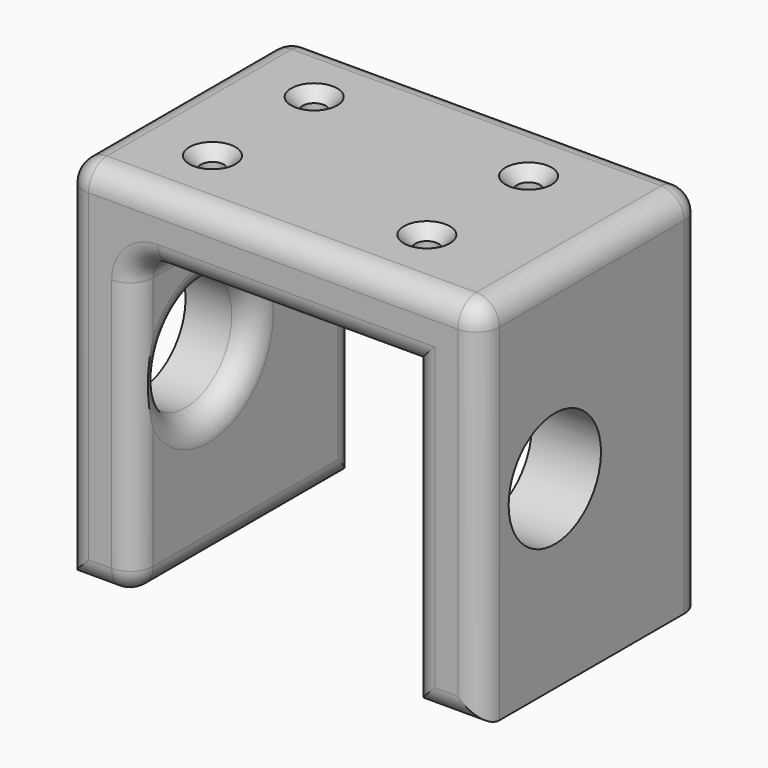
from build123d import *

# Parameters (mm, degrees)
F1_DEPTH       = 38.1
F3_D           = 31.75
F4_T1_DEPTH    = 76.2
F4_T3_DEPTH    = 101.6
F4_T5_DEPTH    = 111.125
F4_T7_DEPTH    = 28.575
F4_T9_DEPTH    = 69.85
F4_T11_DEPTH   = 69.85
F4_T13_DEPTH   = 98.425
F4_T15_DEPTH   = 50.8
F4_T17_DEPTH   = 63.5
F4_T19_DEPTH   = 85.725
F4_T21_DEPTH   = 92.075
F4_S25_W       = 6.477
F4_S25_H       = 6.477
F4_T26_DEPTH   = 6.477
F4_S31_W       = 6.477
F4_S31_H       = 6.477
F4_T32_DEPTH   = 6.477
F4_S37_W       = 6.477
F4_S37_H       = 6.477
F4_T38_DEPTH   = 6.477
F4_S43_W       = 6.477
F4_S43_H       = 6.477
F4_T44_DEPTH   = 6.477
F4_S49_W       = 6.477
F4_S49_H       = 6.477
F4_T50_DEPTH   = 6.477
F4_T56_ANGLE   = 90
F4_T58_ANGLE   = 90
F4_T63_DEPTH   = 85.725
F4_T67_DEPTH   = 98.425
F4_T74_DEPTH   = 85.725
F4_T78_DEPTH   = 98.425
F6_D           = 6.35
F6_DEPTH       = 12.7
F6_CSINK_D     = 12.7
F6_CSINK_ANGLE = 90
F6_TIP         = 1.9077324654


# Not quite as in the source:
# - a fillet or chamfer that OpenCascade refuses, or shapes differently, is made with other operations: its cross-section is extruded or revolved along the edge and cut away or added


with BuildPart() as f1:
    # F0 (on Front) → F1 (new body, symmetric)
    with BuildSketch(Plane.XZ):
        Polygon((57.15, 50.8), (-57.15, 50.8), (-57.15, -50.8), (-38.1, -50.8), (-38.1, 31.75), (38.1, 31.75), (38.1, -50.8), (57.15, -50.8), align=None)
    extrude(amount=F1_DEPTH, both=True)

    # F3 (through all)
    with Locations(Plane.YZ.offset(57.15)):
        with Locations((-12.7, 0)):
            Hole(F3_D / 2)

    # F4: fillet of radius 6.35 on 19 edges, made by hand

    # F4_s2 → F4_t1 (join)
    with BuildSketch(Plane.XZ.offset(-38.1)):
        with BuildLine():
            ThreePointArc((-38.1, 25.4), (-36.2401280605, 29.8901280605), (-31.75, 31.75))
            Line((-31.75, 31.75), (-38.1, 31.75))
            Line((-38.1, 31.75), (-38.1, 25.4))
        make_face()
    extrude(amount=F4_T1_DEPTH)

    # F4_s4 → F4_t3 (cut)
    with BuildSketch(Plane.YZ.offset(-50.8)):
        with BuildLine():
            ThreePointArc((-31.75, 50.8), (-36.2401280605, 48.9401280605), (-38.1, 44.45))
            Line((-38.1, 44.45), (-38.1, 50.8))
            Line((-38.1, 50.8), (-31.75, 50.8))
        make_face()
        with BuildLine():
            ThreePointArc((31.75, 50.8), (36.2401280605, 48.9401280605), (38.1, 44.45))
            Line((38.1, 44.45), (38.1, 50.8))
            Line((38.1, 50.8), (31.75, 50.8))
        make_face()
    extrude(amount=F4_T3_DEPTH, mode=Mode.SUBTRACT)

    # F4_s6 → F4_t5 (cut)
    with BuildSketch(Plane.XY.offset(-66.675)):
        with BuildLine():
            ThreePointArc((-57.15, -31.75), (-55.2901280605, -36.2401280605), (-50.8, -38.1))
            Line((-50.8, -38.1), (-57.15, -38.1))
            Line((-57.15, -38.1), (-57.15, -31.75))
        make_face()
        with BuildLine():
            ThreePointArc((50.8, -38.1), (55.2901280605, -36.2401280605), (57.15, -31.75))
            Line((57.15, -31.75), (57.15, -38.1))
            Line((57.15, -38.1), (50.8, -38.1))
        make_face()
        with BuildLine():
            ThreePointArc((50.8, 38.1), (55.2901280605, 36.2401280605), (57.15, 31.75))
            Line((57.15, 31.75), (57.15, 38.1))
            Line((57.15, 38.1), (50.8, 38.1))
        make_face()
        with BuildLine():
            ThreePointArc((-50.8, 38.1), (-55.2901280605, 36.2401280605), (-57.15, 31.75))
            Line((-57.15, 31.75), (-57.15, 38.1))
            Line((-57.15, 38.1), (-50.8, 38.1))
        make_face()
    extrude(amount=F4_T5_DEPTH, mode=Mode.SUBTRACT)

    # F4_s8 → F4_t7 (cut)
    with BuildSketch(Plane.YZ.offset(-73.025)):
        with BuildLine():
            ThreePointArc((-38.1, -44.45), (-36.2401280605, -48.9401280605), (-31.75, -50.8))
            Line((-31.75, -50.8), (-38.1, -50.8))
            Line((-38.1, -50.8), (-38.1, -44.45))
        make_face()
    extrude(amount=F4_T7_DEPTH, mode=Mode.SUBTRACT)

    # F4_s10 → F4_t9 (cut)
    with BuildSketch(Plane.XY.offset(-44.45)):
        with BuildLine():
            ThreePointArc((-44.45, -38.1), (-39.9598719395, -36.2401280605), (-38.1, -31.75))
            Line((-38.1, -31.75), (-38.1, -38.1))
            Line((-38.1, -38.1), (-44.45, -38.1))
        make_face()
    extrude(amount=F4_T9_DEPTH, mode=Mode.SUBTRACT)

    # F4_s12 → F4_t11 (cut)
    with BuildSketch(Plane.YZ.offset(-31.75)):
        with BuildLine():
            ThreePointArc((-38.1, 38.1), (-36.2401280605, 33.6098719395), (-31.75, 31.75))
            Line((-31.75, 31.75), (-38.1, 31.75))
            Line((-38.1, 31.75), (-38.1, 38.1))
        make_face()
        with BuildLine():
            ThreePointArc((38.1, 38.1), (36.2401280605, 33.6098719395), (31.75, 31.75))
            Line((31.75, 31.75), (38.1, 31.75))
            Line((38.1, 31.75), (38.1, 38.1))
        make_face()
    extrude(amount=F4_T11_DEPTH, mode=Mode.SUBTRACT)

    # F4_s14 → F4_t13 (cut)
    with BuildSketch(Plane.XY.offset(-66.675)):
        with BuildLine():
            ThreePointArc((44.45, -38.1), (39.9598719395, -36.2401280605), (38.1, -31.75))
            Line((38.1, -31.75), (38.1, -38.1))
            Line((38.1, -38.1), (44.45, -38.1))
        make_face()
        with BuildLine():
            ThreePointArc((44.45, 38.1), (39.9598719395, 36.2401280605), (38.1, 31.75))
            Line((38.1, 31.75), (38.1, 38.1))
            Line((38.1, 38.1), (44.45, 38.1))
        make_face()
    extrude(amount=F4_T13_DEPTH, mode=Mode.SUBTRACT)

    # F4_s16 → F4_t15 (cut)
    with BuildSketch(Plane.YZ.offset(22.225)):
        with BuildLine():
            ThreePointArc((-38.1, -44.45), (-36.2401280605, -48.9401280605), (-31.75, -50.8))
            Line((-31.75, -50.8), (-38.1, -50.8))
            Line((-38.1, -50.8), (-38.1, -44.45))
        make_face()
    extrude(amount=F4_T15_DEPTH, mode=Mode.SUBTRACT)

    # F4_s18 → F4_t17 (cut)
    with BuildSketch(Plane.XZ.offset(-31.75)):
        with BuildLine():
            ThreePointArc((-50.8, 50.8), (-55.2901280605, 48.9401280605), (-57.15, 44.45))
            Line((-57.15, 44.45), (-57.15, 50.8))
            Line((-57.15, 50.8), (-50.8, 50.8))
        make_face()
        with BuildLine():
            ThreePointArc((50.8, 50.8), (55.2901280605, 48.9401280605), (57.15, 44.45))
            Line((57.15, 44.45), (57.15, 50.8))
            Line((57.15, 50.8), (50.8, 50.8))
        make_face()
    extrude(amount=F4_T17_DEPTH, mode=Mode.SUBTRACT)

    # F4_s20 → F4_t19 (cut)
    with BuildSketch(Plane.XZ.offset(-53.975)):
        with BuildLine():
            ThreePointArc((-44.45, -50.8), (-39.9598719395, -48.9401280605), (-38.1, -44.45))
            Line((-38.1, -44.45), (-38.1, -50.8))
            Line((-38.1, -50.8), (-44.45, -50.8))
        make_face()
    extrude(amount=F4_T19_DEPTH, mode=Mode.SUBTRACT)

    # F4_s22 → F4_t21 (cut)
    with BuildSketch(Plane.XY.offset(-66.675)):
        with BuildLine():
            ThreePointArc((-44.45, 38.1), (-39.9598719395, 36.2401280605), (-38.1, 31.75))
            Line((-38.1, 31.75), (-38.1, 38.1))
            Line((-38.1, 38.1), (-44.45, 38.1))
        make_face()
    extrude(amount=F4_T21_DEPTH, mode=Mode.SUBTRACT)


with BuildPart() as f4_tool24:
    # F4_s25 → F4_t26 (new body)
    with BuildSketch(Plane.XY.offset(44.45)):
        with Locations((54.0385, -34.9885)):
            Rectangle(F4_S25_W, F4_S25_H)
    extrude(amount=F4_T26_DEPTH)

    # F4_s27 → F4_t28 (revolve, cut)
    with BuildSketch(Plane(origin=(50.8, -31.75, 44.45), x_dir=(-0.7071067812, 0.7071067812, 0), z_dir=(0.7071067812, 0.7071067812, 0))):
        with BuildLine():
            ThreePointArc((0, -6.35), (6.35, 0), (0, 6.35))
            Line((0, 6.35), (0, -6.35))
        make_face()
    revolve(axis=Axis((50.8, -31.75, 44.45), (0, 0, 1)), mode=Mode.SUBTRACT)


with BuildPart() as f1_1:
    add(f1.part)

    # F4_t23: cut F4_tool24
    add(f4_tool24.part, mode=Mode.SUBTRACT)


with BuildPart() as f4_tool30:
    # F4_s31 → F4_t32 (new body)
    with BuildSketch(Plane.XY.offset(44.45)):
        with Locations((-54.0385, -34.9885)):
            Rectangle(F4_S31_W, F4_S31_H)
    extrude(amount=F4_T32_DEPTH)

    # F4_s33 → F4_t34 (revolve, cut)
    with BuildSketch(Plane(origin=(-50.8, -31.75, 44.45), x_dir=(0.7071067812, 0.7071067812, 0), z_dir=(0.7071067812, -0.7071067812, 0))):
        with BuildLine():
            ThreePointArc((0, -6.35), (6.35, 0), (0, 6.35))
            Line((0, 6.35), (0, -6.35))
        make_face()
    revolve(axis=Axis((-50.8, -31.75, 44.45), (0, 0, 1)), mode=Mode.SUBTRACT)


with BuildPart() as f1_2:
    add(f1_1.part)

    # F4_t29: cut F4_tool30
    add(f4_tool30.part, mode=Mode.SUBTRACT)


with BuildPart() as f4_tool36:
    # F4_s37 → F4_t38 (new body)
    with BuildSketch(Plane.XZ.offset(31.75)):
        with Locations((-41.2115, -47.6885)):
            Rectangle(F4_S37_W, F4_S37_H)
    extrude(amount=F4_T38_DEPTH)

    # F4_s39 → F4_t40 (revolve, cut)
    with BuildSketch(Plane(origin=(-44.45, -31.75, -44.45), x_dir=(-0.7071067812, 0, 0.7071067812), z_dir=(0.7071067812, 0, 0.7071067812))):
        with BuildLine():
            ThreePointArc((0, -6.35), (6.35, 0), (0, 6.35))
            Line((0, 6.35), (0, -6.35))
        make_face()
    revolve(axis=Axis((-44.45, -31.75, -44.45), (0, -1, 0)), mode=Mode.SUBTRACT)


with BuildPart() as f1_3:
    add(f1_2.part)

    # F4_t35: cut F4_tool36
    add(f4_tool36.part, mode=Mode.SUBTRACT)


with BuildPart() as f4_tool42:
    # F4_s43 → F4_t44 (new body)
    with BuildSketch(Plane.XY.offset(44.45)):
        with Locations((-54.0385, 34.9885)):
            Rectangle(F4_S43_W, F4_S43_H)
    extrude(amount=F4_T44_DEPTH)

    # F4_s45 → F4_t46 (revolve, cut)
    with BuildSketch(Plane(origin=(-50.8, 31.75, 44.45), x_dir=(0.7071067812, -0.7071067812, 0), z_dir=(-0.7071067812, -0.7071067812, 0))):
        with BuildLine():
            ThreePointArc((0, -6.35), (6.35, 0), (0, 6.35))
            Line((0, 6.35), (0, -6.35))
        make_face()
    revolve(axis=Axis((-50.8, 31.75, 44.45), (0, 0, 1)), mode=Mode.SUBTRACT)


with BuildPart() as f1_4:
    add(f1_3.part)

    # F4_t41: cut F4_tool42
    add(f4_tool42.part, mode=Mode.SUBTRACT)


with BuildPart() as f4_tool48:
    # F4_s49 → F4_t50 (new body)
    with BuildSketch(Plane.XY.offset(44.45)):
        with Locations((54.0385, 34.9885)):
            Rectangle(F4_S49_W, F4_S49_H)
    extrude(amount=F4_T50_DEPTH)

    # F4_s51 → F4_t52 (revolve, cut)
    with BuildSketch(Plane(origin=(50.8, 31.75, 44.45), x_dir=(-0.7071067812, -0.7071067812, 0), z_dir=(-0.7071067812, 0.7071067812, 0))):
        with BuildLine():
            ThreePointArc((0, -6.35), (6.35, 0), (0, 6.35))
            Line((0, 6.35), (0, -6.35))
        make_face()
    revolve(axis=Axis((50.8, 31.75, 44.45), (0, 0, 1)), mode=Mode.SUBTRACT)


with BuildPart() as f1_5:
    add(f1_4.part)

    # F4_t47: cut F4_tool48
    add(f4_tool48.part, mode=Mode.SUBTRACT)

    # F4_s53 → F4_t54 (revolve, cut)
    with BuildSketch(Plane.XY):
        with BuildLine():
            ThreePointArc((-38.1, 9.525), (-39.9598719395, 5.0348719395), (-44.45, 3.175))
            Line((-44.45, 3.175), (-38.1, 3.175))
            Line((-38.1, 3.175), (-38.1, 9.525))
        make_face()
    revolve(axis=Axis((-38.1, -12.7, 0), (1, 0, 0)), mode=Mode.SUBTRACT)

    # F4_s55 → F4_t56 (revolve, cut)
    with BuildSketch(Plane.XY.offset(25.4)):
        with BuildLine():
            ThreePointArc((-44.45, 38.1), (-39.9598719395, 36.2401280605), (-38.1, 31.75))
            Line((-38.1, 31.75), (-38.1, 38.1))
            Line((-38.1, 38.1), (-44.45, 38.1))
        make_face()
    revolve(axis=Axis((-31.75, 38.1, 25.4), (0, 1, 0)), revolution_arc=F4_T56_ANGLE, mode=Mode.SUBTRACT)

    # F4_s57 → F4_t58 (revolve, cut)
    with BuildSketch(Plane.XY.offset(25.4)):
        with BuildLine():
            ThreePointArc((-44.45, -38.1), (-39.9598719395, -36.2401280605), (-38.1, -31.75))
            Line((-38.1, -31.75), (-38.1, -38.1))
            Line((-38.1, -38.1), (-44.45, -38.1))
        make_face()
    revolve(axis=Axis((-31.75, -38.1, 25.4), (0, 1, 0)), revolution_arc=F4_T58_ANGLE, mode=Mode.SUBTRACT)


with BuildPart() as f4_tool61:
    # F4_s62 → F4_t63 (new body)
    with BuildSketch(Plane.YZ.offset(-31.75)):
        with BuildLine():
            ThreePointArc((-38.1, 38.1), (-36.2401280605, 33.6098719395), (-31.75, 31.75))
            Line((-31.75, 31.75), (-38.1, 31.75))
            Line((-38.1, 31.75), (-38.1, 38.1))
        make_face()
    extrude(amount=F4_T63_DEPTH)

    split(bisect_by=Plane.YZ.offset(38.1), keep=Keep.TOP)


with BuildPart() as f4_tool65:
    # F4_s66 → F4_t67 (new body)
    with BuildSketch(Plane.XY.offset(47.625)):
        with BuildLine():
            ThreePointArc((44.45, -38.1), (39.9598719395, -36.2401280605), (38.1, -31.75))
            Line((38.1, -31.75), (38.1, -38.1))
            Line((38.1, -38.1), (44.45, -38.1))
        make_face()
    extrude(amount=-F4_T67_DEPTH)

    split(bisect_by=Plane.XY.offset(31.75), keep=Keep.TOP)


with BuildPart() as f4_tool61_1:
    add(f4_tool61.part)

    # F4_t69: intersect F4_tool65
    add(f4_tool65.part, mode=Mode.INTERSECT)


with BuildPart() as f1_6:
    add(f1_5.part)

    # F4_t59: cut F4_tool61
    add(f4_tool61_1.part, mode=Mode.SUBTRACT)


with BuildPart() as f4_tool72:
    # F4_s73 → F4_t74 (new body)
    with BuildSketch(Plane.YZ.offset(-31.75)):
        with BuildLine():
            ThreePointArc((38.1, 38.1), (36.2401280605, 33.6098719395), (31.75, 31.75))
            Line((31.75, 31.75), (38.1, 31.75))
            Line((38.1, 31.75), (38.1, 38.1))
        make_face()
    extrude(amount=F4_T74_DEPTH)

    split(bisect_by=Plane.YZ.offset(38.1), keep=Keep.TOP)


with BuildPart() as f4_tool76:
    # F4_s77 → F4_t78 (new body)
    with BuildSketch(Plane.XY.offset(47.625)):
        with BuildLine():
            ThreePointArc((44.45, 38.1), (39.9598719395, 36.2401280605), (38.1, 31.75))
            Line((38.1, 31.75), (38.1, 38.1))
            Line((38.1, 38.1), (44.45, 38.1))
        make_face()
    extrude(amount=-F4_T78_DEPTH)

    split(bisect_by=Plane.XY.offset(31.75), keep=Keep.TOP)


with BuildPart() as f4_tool72_1:
    add(f4_tool72.part)

    # F4_t80: intersect F4_tool76
    add(f4_tool76.part, mode=Mode.INTERSECT)


with BuildPart() as f1_7:
    add(f1_6.part)

    # F4_t70: cut F4_tool72
    add(f4_tool72_1.part, mode=Mode.SUBTRACT)

    # F6
    with Locations(Plane.XY.offset(50.8)):
        with Locations((-33.2249589264, 17.5176411867), (25.7616862655, 17.5176411867), (25.7616862655, -17.4796506763), (-33.2249589264, -17.4796506763)):
            CounterSinkHole(F6_D / 2, F6_CSINK_D / 2, depth=F6_DEPTH, counter_sink_angle=F6_CSINK_ANGLE)
            with Locations((0, 0, -(F6_DEPTH + F6_TIP / 2))):  # 118° drill point
                Cone(0, F6_D / 2, F6_TIP, mode=Mode.SUBTRACT)


solid = f1_7.part
